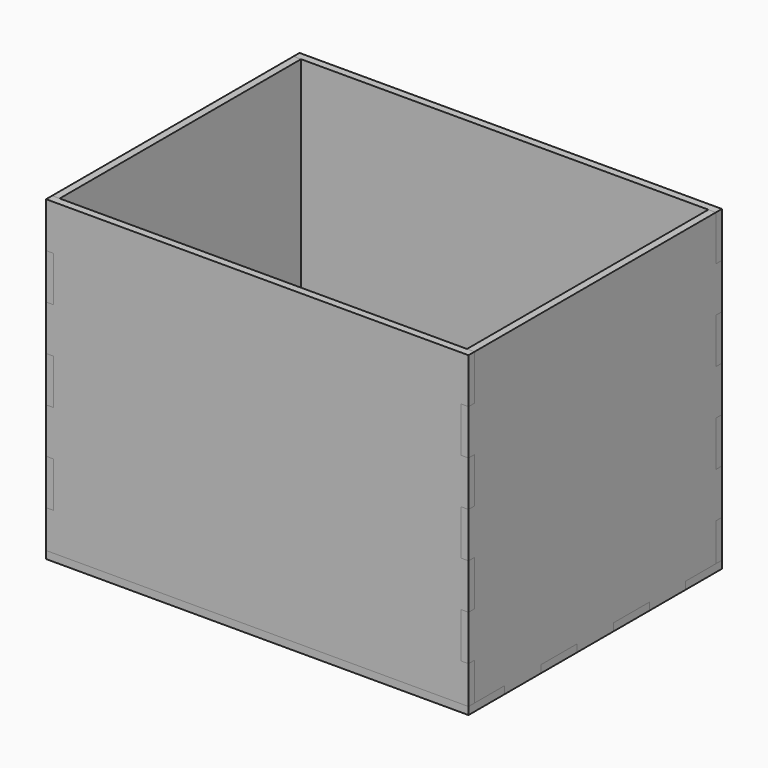
from build123d import *

# Parameters (mm, degrees)
F0_W      = 177.8
F0_H      = 133.35
F1_DEPTH  = 3.175
F2_W      = 3.175
F2_H      = 133.35
F3_DEPTH  = 133.35
F4_W      = 19.05
F4_H      = 3.175
F5_DEPTH  = 3.175
F6_W      = 177.8
F6_H      = 130.175
F7_DEPTH  = 3.175
F8_W      = 3.175
F8_H      = 19.05
F9_DEPTH  = 3.175
F11_COUNT = 2
F11_ANGLE = 180


with BuildPart() as f1:
    # F0 (on Top) → F1 (new body)
    with BuildSketch(Plane.XY):
        Rectangle(F0_W, F0_H)
    extrude(amount=F1_DEPTH)


with BuildPart() as f3:
    # F2 (on face) → F3 (new body)
    with BuildSketch(Plane(origin=(0, 0, 0), x_dir=(1, 0, 0), z_dir=(0, 0, -1))):
        with Locations((87.3125, 0)):
            Rectangle(F2_W, F2_H)
    extrude(amount=-F3_DEPTH)

    # F4 (on face) → F5 (cut)
    with BuildSketch(Plane.YZ.offset(88.9)):
        with Locations((-57.15, 1.5875)):
            Rectangle(F4_W, F4_H)
        with Locations((-19.05, 1.5875)):
            Rectangle(F4_W, F4_H)
        with Locations((19.05, 1.5875)):
            Rectangle(F4_W, F4_H)
        with Locations((57.15, 1.5875)):
            Rectangle(F4_W, F4_H)
    extrude(amount=-F5_DEPTH, mode=Mode.SUBTRACT)

    # F8 (on face) → F9 (cut)
    with BuildSketch(Plane.YZ.offset(88.9)):
        with Locations((65.0875, 123.825)):
            Rectangle(F8_W, F8_H)
        with Locations((65.0875, 85.725)):
            Rectangle(F8_W, F8_H)
        with Locations((65.0875, 47.625)):
            Rectangle(F8_W, F8_H)
        with Locations((65.0875, 9.525)):
            Rectangle(F8_W, F8_H)
        with Locations((-65.0875, 123.825)):
            Rectangle(F8_W, F8_H)
        with Locations((-65.0875, 85.725)):
            Rectangle(F8_W, F8_H)
        with Locations((-65.0875, 47.625)):
            Rectangle(F8_W, F8_H)
        with Locations((-65.0875, 9.525)):
            Rectangle(F8_W, F8_H)
    extrude(amount=-F9_DEPTH, mode=Mode.SUBTRACT)


with BuildPart() as f7:
    # F6 (on face) → F7 (new body)
    with BuildSketch(Plane(origin=(0, 66.675, 0), x_dir=(-1, 0, 0), z_dir=(0, 1, 0))):
        with Locations((0, 68.2625)):
            Rectangle(F6_W, F6_H)
    extrude(amount=-F7_DEPTH)


with BuildPart() as f11_1:
    # F11: instance of F7
    add(f7.part.rotate(Axis((0, 0, 37.3618602753), (0, 0, -1)), 1 * F11_ANGLE / (F11_COUNT - 1)))


with BuildPart() as f11_2:
    # F11: instance of F3
    add(f3.part.rotate(Axis((0, 0, 37.3618602753), (0, 0, -1)), 1 * F11_ANGLE / (F11_COUNT - 1)))


with BuildPart() as f1_1:
    add(f1.part)

    # F12: cut F3, F11_2
    add(f3.part, mode=Mode.SUBTRACT)
    add(f11_2.part, mode=Mode.SUBTRACT)


with BuildPart() as f7_1:
    add(f7.part)

    # F12: cut F3, F11_2
    add(f3.part, mode=Mode.SUBTRACT)
    add(f11_2.part, mode=Mode.SUBTRACT)


with BuildPart() as f11_1_1:
    add(f11_1.part)

    # F12: cut F3, F11_2
    add(f3.part, mode=Mode.SUBTRACT)
    add(f11_2.part, mode=Mode.SUBTRACT)


solid = Compound([f3.part, f11_2.part, f1_1.part, f7_1.part, f11_1_1.part])
